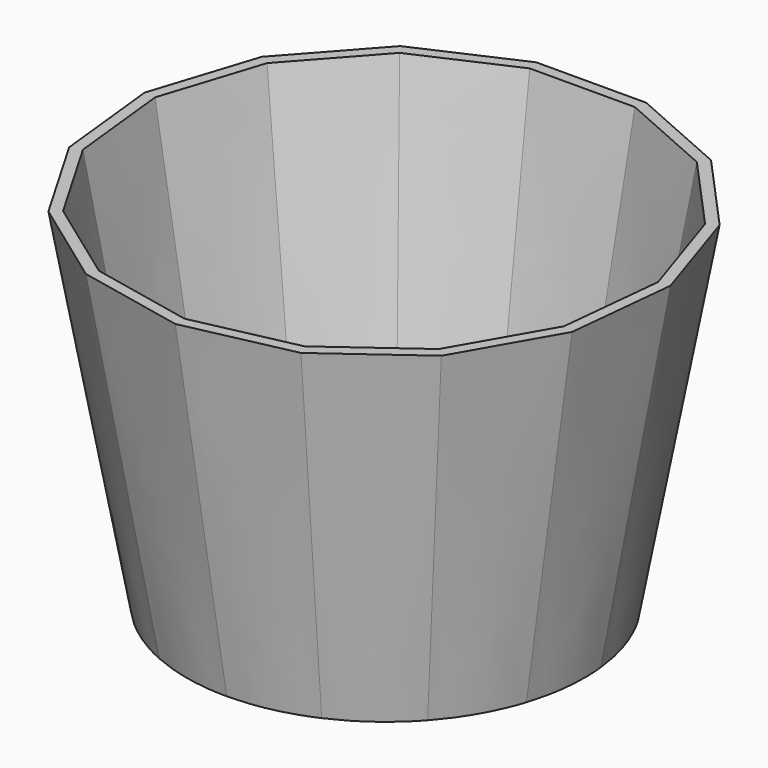
from build123d import *

# Parameters (mm, degrees)
F5_T            = 2.5
F6_R            = 35
F7_DEPTH        = 5
F8_R            = 1.55
F9_DEPTH        = 5
F9_COPIES_COUNT = 4


# Not quite as in the source:
# - the arcs of a loft's sections are written as splines that run evenly, so that the points pair up as in the source's solid
# - a pattern or mirror of a feature is missing from the dataset's text; its kind, count and spacing are read off the source's solid
# - a shell that OpenCascade refuses in one call is made with other operations: the cavity is built on its own and cut out


with BuildPart() as f4:
    # F0 (on Top) → F4 section 0
    with BuildSketch(Plane.XY):
        with BuildLine():
            add(Edge.make_bspline(
                [(42.8369797645, -13.7838008059), (43.7992705945, -10.7932154519), (44.4472175017, -7.7015881973), (45.0861871199, -1.4509773926), (45.0771893826, 1.7078061259), (44.7399051516, 4.8312407336)],
                knots=[0, 0, 0, 0, 0.5, 0.5, 1, 1, 1, 1], degree=3))
            add(Edge.make_bspline(
                [(44.7399051516, 4.8312407336), (44.4026209206, 7.9546753413), (43.7370717832, 11.0425611265), (41.7784471196, 17.0126705921), (40.4854342731, 19.8947032177), (38.9068944887, 22.6109168599)],
                knots=[0, 0, 0, 0, 0.5, 0.5, 1, 1, 1, 1], degree=3))
            add(Edge.make_bspline(
                [(38.9068944887, 22.6109168599), (37.3283547043, 25.3271305021), (35.4643890146, 27.8773513129), (31.2468340671, 32.5346732761), (28.8933797791, 34.6416253854), (26.3465283107, 36.4809600473)],
                knots=[0, 0, 0, 0, 0.5, 0.5, 1, 1, 1, 1], degree=3))
            add(Edge.make_bspline(
                [(26.3465283107, 36.4809600473), (23.7996768422, 38.3202947093), (21.0595912015, 39.8918941995), (15.3123595358, 42.4311353825), (12.3053974332, 43.3986958146), (9.230608037, 44.0431138235)],
                knots=[0, 0, 0, 0, 0.5, 0.5, 1, 1, 1, 1], degree=3))
            add(Edge.make_bspline(
                [(9.230608037, 44.0431138235), (6.1558186408, 44.6875318323), (3.0133987493, 45.0087661726), (-3.2697610676, 44.9908687065), (-6.4102999199, 44.6517374728), (-9.4813682236, 43.9898131004)],
                knots=[0, 0, 0, 0, 0.5, 0.5, 1, 1, 1, 1], degree=3))
            add(Edge.make_bspline(
                [(-9.4813682236, 43.9898131004), (-12.5524365274, 43.327888728), (-15.5538377225, 42.3432135826), (-21.2865102776, 39.7712721019), (-24.0175981811, 38.1840880736), (-26.5539297829, 36.3302740574)],
                knots=[0, 0, 0, 0, 0.5, 0.5, 1, 1, 1, 1], degree=3))
            add(Edge.make_bspline(
                [(-26.5539297829, 36.3302740574), (-29.0902613847, 34.4764600411), (-31.43167435, 32.3561346882), (-35.6226284788, 27.6748612402), (-37.4720355238, 25.1140629549), (-39.0350756479, 22.3889005796)],
                knots=[0, 0, 0, 0, 0.5, 0.5, 1, 1, 1, 1], degree=3))
            add(Edge.make_bspline(
                [(-39.0350756479, 22.3889005796), (-40.5981157719, 19.6637382044), (-41.8746889345, 16.7743861599), (-43.7992705945, 10.7932154519), (-44.4472175017, 7.7015881973), (-44.7667023108, 4.5762827949)],
                knots=[0, 0, 0, 0, 0.5, 0.5, 1, 1, 1, 1], degree=3))
            add(Edge.make_bspline(
                [(-44.7667023108, 4.5762827949), (-45.0861871199, 1.4509773926), (-45.0771893826, -1.7078061259), (-44.4026209206, -7.9546753413), (-43.7370717832, -11.0425611265), (-42.7577594514, -14.0276158593)],
                knots=[0, 0, 0, 0, 0.5, 0.5, 1, 1, 1, 1], degree=3))
            add(Edge.make_bspline(
                [(-42.7577594514, -14.0276158593), (-41.7784471196, -17.0126705921), (-40.4854342731, -19.8947032177), (-37.3283547043, -25.3271305021), (-35.4643890146, -27.8773513129), (-33.3556115409, -30.2060122945)],
                knots=[0, 0, 0, 0, 0.5, 0.5, 1, 1, 1, 1], degree=3))
            add(Edge.make_bspline(
                [(-33.3556115409, -30.2060122945), (-31.2468340671, -32.5346732761), (-28.8933797791, -34.6416253854), (-23.7996768422, -38.3202947093), (-21.0595912015, -39.8918941995), (-18.1859753687, -41.161514791)],
                knots=[0, 0, 0, 0, 0.5, 0.5, 1, 1, 1, 1], degree=3))
            add(Edge.make_bspline(
                [(-18.1859753687, -41.161514791), (-15.3123595358, -42.4311353825), (-12.3053974332, -43.3986958146), (-6.1558186408, -44.6875318323), (-3.0133987493, -45.0087661726), (0.1281811592, -44.9998174395)],
                knots=[0, 0, 0, 0, 0.5, 0.5, 1, 1, 1, 1], degree=3))
            add(Edge.make_bspline(
                [(0.1281811592, -44.9998174395), (3.2697610676, -44.9908687065), (6.4102999199, -44.6517374728), (12.5524365274, -43.327888728), (15.5538377225, -42.3432135826), (18.4201740001, -41.0572428422)],
                knots=[0, 0, 0, 0, 0.5, 0.5, 1, 1, 1, 1], degree=3))
            add(Edge.make_bspline(
                [(18.4201740001, -41.0572428422), (21.2865102776, -39.7712721019), (24.0175981811, -38.1840880736), (29.0902613847, -34.4764600411), (31.43167435, -32.3561346882), (33.5271514144, -30.0154979642)],
                knots=[0, 0, 0, 0, 0.5, 0.5, 1, 1, 1, 1], degree=3))
            add(Edge.make_bspline(
                [(33.5271514144, -30.0154979642), (35.6226284788, -27.6748612402), (37.4720355238, -25.1140629549), (40.5981157719, -19.6637382044), (41.8746889345, -16.7743861599), (42.8369797645, -13.7838008059)],
                knots=[0, 0, 0, 0, 0.5, 0.5, 1, 1, 1, 1], degree=3))
        make_face()
    # F3 (on offset) → F4 section 1
    with BuildSketch(Plane.XY.offset(80)):
        Polygon((56.727516118, -18.253405975), (59.2474937439, 6.3978433609), (51.5230414549, 29.9428474571), (34.8897872262, 48.3104612057), (12.2237718224, 58.3247573252), (-12.5558447791, 58.2541730393), (-35.1644417519, 48.1109130123), (-51.692787287, 29.6488390516), (-59.2829802858, 6.0602114677), (-56.6226074243, -18.5762817343), (-44.1716713389, -40.0007670643), (-24.083051992, -54.5087563732), (0.169745832, -59.5916865087), (24.3931930596, -54.3706726734), (44.398835602, -39.7484755908), align=None)
    loft(ruled=True)

    # F5: shell of thickness 2.5, made by hand


with BuildPart() as f5_core1:
    # F5_t2: copy of F4
    add(f4.part)

    # the walls: a layer under each face that stays
    f5_faces = [f5_core1.faces().sort_by_distance(p)[0] for p in [
        (10.8814188347, -50.4854963457, 40),
        (30.4749720569, -41.6949240947, 40),
        (44.7991257539, -25.6949206813, 40),
        (51.3771036209, -5.252032051, 40),
        (49.0715135254, 16.0989806341, 40),
        (38.2810129407, 34.666333313, 40),
        (20.8713774465, 47.2395620282, 40),
        (-0.1471088188, 51.6446413109, 40),
        (-21.1401586328, 47.119892934, 40),
        (-38.4778829669, 34.4476869981, 40),
        (-49.1624317754, 15.8191630328, 40),
        (-51.3463495033, -5.5446379335, 40),
        (-44.6520169352, -25.9497206296, 40),
        (-30.2369449881, -41.867860883, 40),
        (-10.5936305585, -50.5466676322, 40),
        (0, 0, 0),
    ]]
    thicken(f5_faces, amount=-F5_T, mode=Mode.SUBTRACT)


with BuildPart() as f4_1:
    add(f4.part)

    # what is left inside the walls is the cavity
    f5_cavity = [f5_core1.part.solids().sort_by_distance(p)[0] for p in [
        (-18.066543, -1.950916, 79.975),
    ]]
    add(f5_cavity, mode=Mode.SUBTRACT)

    # F6 (on face) → F7 (cut)
    with BuildSketch(Plane.XY):
        Circle(F6_R)
    extrude(amount=F7_DEPTH, mode=Mode.SUBTRACT)

    # F8 (on Top) → F9 (cut)
    with BuildSketch(Plane.XY):
        with Locations((-39.5, 0)):
            Circle(F8_R)
    f9 = extrude(amount=F9_DEPTH, mode=Mode.SUBTRACT)

    # F9_copies: F9 ×4 about axis
    f9_copies_axis = Axis((0, 0, 0), (0, 0, 1))
    for i in range(1, F9_COPIES_COUNT):
        add(f9.rotate(f9_copies_axis, i * 360 / F9_COPIES_COUNT), mode=Mode.SUBTRACT)


solid = f4_1.part
